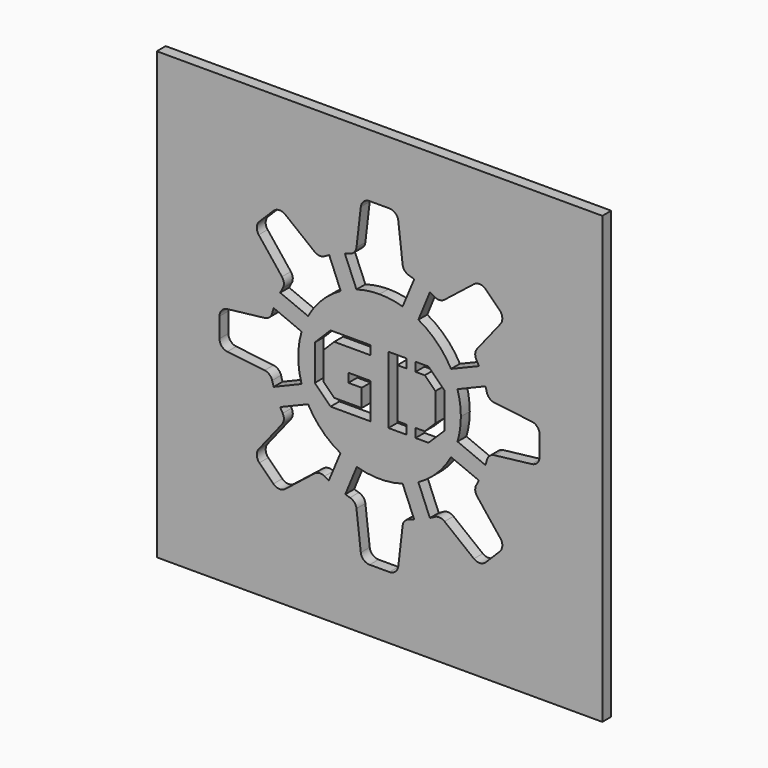
from build123d import *

# Parameters (mm, degrees)
F0_W     = 127
F0_H     = 127
F1_DEPTH = 3.175
F3_DEPTH = 3.175
F5_DEPTH = 3.175
F7_DEPTH = 3.175


with BuildPart() as f1:
    # F0 (on Front) → F1 (new body)
    with BuildSketch(Plane.XZ):
        Rectangle(F0_W, F0_H)
    extrude(amount=-F1_DEPTH)

    # F2 (on face) → F3 (cut, through all)
    with BuildSketch(Plane.XZ):
        with BuildLine():
            ThreePointArc((-6.5756926955, 32.7672866468), (-7.1708300148, 31.407037356), (-8.424698119, 30.611876153))
            ThreePointArc((-8.424698119, 30.611876153), (-12.1501989776, 29.3331751572), (-15.6887040432, 27.603026382))
            ThreePointArc((-15.6887040432, 27.603026382), (-17.1375865613, 27.2786716216), (-18.520253693, 27.819687485))
            Line((-18.520253693, 27.819687485), (-26.8947926181, 34.4486268529))
            ThreePointArc((-26.8947926181, 34.4486268529), (-28.6182622131, 34.9927875941), (-30.2672971687, 34.2530970695))
            Line((-30.2672971687, 34.2530970695), (-32.2601971191, 32.2601971191))
            Line((-32.2601971191, 32.2601971191), (-34.2530970695, 30.2672971687))
            ThreePointArc((-34.2530970695, 30.2672971687), (-34.9927875941, 28.6182622131), (-34.4486268529, 26.8947926181))
            Line((-34.4486268529, 26.8947926181), (-27.819687485, 18.520253693))
            ThreePointArc((-27.819687485, 18.520253693), (-27.2786716216, 17.1375865613), (-27.603026382, 15.6887040432))
            ThreePointArc((-27.603026382, 15.6887040432), (-29.3331751572, 12.1501989776), (-30.611876153, 8.424698119))
            ThreePointArc((-30.611876153, 8.424698119), (-31.407037356, 7.1708300148), (-32.7672866468, 6.5756926955))
            Line((-32.7672866468, 6.5756926955), (-43.3763478891, 5.3413674113))
            ThreePointArc((-43.3763478891, 5.3413674113), (-44.9798046771, 4.5074701238), (-45.6228082907, 2.8183861383))
            Line((-45.6228082907, 2.8183861383), (-45.6228082907, 0))
            Line((-45.6228082907, 0), (-45.6228082907, -2.8183861383))
            ThreePointArc((-45.6228082907, -2.8183861383), (-44.9798046771, -4.5074701238), (-43.3763478891, -5.3413674113))
            Line((-43.3763478891, -5.3413674113), (-32.7672866468, -6.5756926955))
            ThreePointArc((-32.7672866468, -6.5756926955), (-31.407037356, -7.1708300148), (-30.611876153, -8.424698119))
            ThreePointArc((-30.611876153, -8.424698119), (-29.3331751572, -12.1501989776), (-27.603026382, -15.6887040432))
            ThreePointArc((-27.603026382, -15.6887040432), (-27.2786716216, -17.1375865613), (-27.819687485, -18.520253693))
            Line((-27.819687485, -18.520253693), (-34.4486268529, -26.8947926181))
            ThreePointArc((-34.4486268529, -26.8947926181), (-34.9927875941, -28.6182622131), (-34.2530970695, -30.2672971687))
            Line((-34.2530970695, -30.2672971687), (-32.2601971191, -32.2601971191))
            Line((-32.2601971191, -32.2601971191), (-30.2672971687, -34.2530970695))
            ThreePointArc((-30.2672971687, -34.2530970695), (-28.6182622131, -34.9927875941), (-26.8947926181, -34.4486268529))
            Line((-26.8947926181, -34.4486268529), (-18.520253693, -27.819687485))
            ThreePointArc((-18.520253693, -27.819687485), (-17.1375865613, -27.2786716216), (-15.6887040432, -27.603026382))
            ThreePointArc((-15.6887040432, -27.603026382), (-15.0740522826, -27.9434329992), (-14.452018381, -28.2701550175))
            Line((-14.452018381, -28.2701550175), (-11.1423706298, -20.3234859952))
            ThreePointArc((-11.1423706298, -20.3234859952), (-22.452662458, 5.7510394537), (0, 23.1775))
            Line((0, 23.1775), (0, 45.6228082907))
            Line((0, 45.6228082907), (-2.8183861383, 45.6228082907))
            ThreePointArc((-2.8183861383, 45.6228082907), (-4.5074701238, 44.9798046771), (-5.3413674113, 43.3763478891))
            Line((-5.3413674113, 43.3763478891), (-6.5756926955, 32.7672866468))
        make_face()
        with BuildLine():
            Line((2.8183861383, 45.6228082907), (0, 45.6228082907))
            Line((0, 45.6228082907), (0, 23.1775))
            ThreePointArc((0, 23.1775), (3.3233858671, 22.9379949566), (6.578087219, 22.2244296842))
            Line((6.578087219, 22.2244296842), (9.8877349702, 30.1710987065))
            ThreePointArc((9.8877349702, 30.1710987065), (9.1588685219, 30.4002899229), (8.424698119, 30.611876153))
            ThreePointArc((8.424698119, 30.611876153), (7.1708300148, 31.407037356), (6.5756926955, 32.7672866468))
            Line((6.5756926955, 32.7672866468), (5.3413674113, 43.3763478891))
            ThreePointArc((5.3413674113, 43.3763478891), (4.5074701238, 44.9798046771), (2.8183861383, 45.6228082907))
        make_face()
        with BuildLine():
            Line((9.8877349702, 30.1710987065), (6.578087219, 22.2244296842))
            ThreePointArc((6.578087219, 22.2244296842), (7.7345087621, 21.8488873964), (8.8696452536, 21.4132178648))
            Line((8.8696452536, 21.4132178648), (12.1501989776, 29.3331751572))
            ThreePointArc((12.1501989776, 29.3331751572), (11.0269289533, 29.7736349454), (9.8877349702, 30.1710987065))
        make_face()
        with BuildLine():
            ThreePointArc((-8.8696452536, -21.4132178648), (-10.0208319922, -20.8992687057), (-11.1423706298, -20.3234859952))
            Line((-11.1423706298, -20.3234859952), (-14.452018381, -28.2701550175))
            ThreePointArc((-14.452018381, -28.2701550175), (-13.31172397, -28.8246509944), (-12.1501989776, -29.3331751572))
            Line((-12.1501989776, -29.3331751572), (-8.8696452536, -21.4132178648))
        make_face()
        with BuildLine():
            Line((12.1501989776, 29.3331751572), (8.8696452536, 21.4132178648))
            ThreePointArc((8.8696452536, 21.4132178648), (9.9803728445, 20.9186200342), (11.0636348579, 20.3664550175))
            Line((11.0636348579, 20.3664550175), (14.3425040432, 28.3258729393))
            ThreePointArc((14.3425040432, 28.3258729393), (13.2559229319, 28.850355409), (12.1501989776, 29.3331751572))
        make_face()
        with BuildLine():
            ThreePointArc((-6.4920289337, -22.2497205954), (-7.6922163688, -21.8638128785), (-8.8696452536, -21.4132178648))
            Line((-8.8696452536, -21.4132178648), (-12.1501989776, -29.3331751572))
            ThreePointArc((-12.1501989776, -29.3331751572), (-10.969295895, -29.7949164719), (-9.770898119, -30.2091385171))
            Line((-9.770898119, -30.2091385171), (-6.4920289337, -22.2497205954))
        make_face()
        with BuildLine():
            Line((14.3425040432, 28.3258729393), (11.0636348579, 20.3664550175))
            ThreePointArc((11.0636348579, 20.3664550175), (19.9201393465, 11.8483988228), (23.1775, 0))
            ThreePointArc((23.1775, 0), (13.9055295771, -18.5427277775), (-6.4920289337, -22.2497205954))
            Line((-6.4920289337, -22.2497205954), (-9.770898119, -30.2091385171))
            ThreePointArc((-9.770898119, -30.2091385171), (-9.1000263744, -30.4179555524), (-8.424698119, -30.611876153))
            ThreePointArc((-8.424698119, -30.611876153), (-7.1708300148, -31.407037356), (-6.5756926955, -32.7672866468))
            Line((-6.5756926955, -32.7672866468), (-5.3413674113, -43.3763478891))
            ThreePointArc((-5.3413674113, -43.3763478891), (-4.5074701238, -44.9798046771), (-2.8183861383, -45.6228082907))
            Line((-2.8183861383, -45.6228082907), (0, -45.6228082907))
            Line((0, -45.6228082907), (2.8183861383, -45.6228082907))
            ThreePointArc((2.8183861383, -45.6228082907), (4.5074701238, -44.9798046771), (5.3413674113, -43.3763478891))
            Line((5.3413674113, -43.3763478891), (6.5756926955, -32.7672866468))
            ThreePointArc((6.5756926955, -32.7672866468), (7.1708300148, -31.407037356), (8.424698119, -30.611876153))
            ThreePointArc((8.424698119, -30.611876153), (12.1501989776, -29.3331751572), (15.6887040432, -27.603026382))
            ThreePointArc((15.6887040432, -27.603026382), (17.1375865613, -27.2786716216), (18.520253693, -27.819687485))
            Line((18.520253693, -27.819687485), (26.8947926181, -34.4486268529))
            ThreePointArc((26.8947926181, -34.4486268529), (28.6182622131, -34.9927875941), (30.2672971687, -34.2530970695))
            Line((30.2672971687, -34.2530970695), (32.2601971191, -32.2601971191))
            Line((32.2601971191, -32.2601971191), (34.2530970695, -30.2672971687))
            ThreePointArc((34.2530970695, -30.2672971687), (34.9927875941, -28.6182622131), (34.4486268529, -26.8947926181))
            Line((34.4486268529, -26.8947926181), (27.819687485, -18.520253693))
            ThreePointArc((27.819687485, -18.520253693), (27.2786716216, -17.1375865613), (27.603026382, -15.6887040432))
            ThreePointArc((27.603026382, -15.6887040432), (29.3331751572, -12.1501989776), (30.611876153, -8.424698119))
            ThreePointArc((30.611876153, -8.424698119), (31.407037356, -7.1708300148), (32.7672866468, -6.5756926955))
            Line((32.7672866468, -6.5756926955), (43.3763478891, -5.3413674113))
            ThreePointArc((43.3763478891, -5.3413674113), (44.9798046771, -4.5074701238), (45.6228082907, -2.8183861383))
            Line((45.6228082907, -2.8183861383), (45.6228082907, 0))
            Line((45.6228082907, 0), (45.6228082907, 2.8183861383))
            ThreePointArc((45.6228082907, 2.8183861383), (44.9798046771, 4.5074701238), (43.3763478891, 5.3413674113))
            Line((43.3763478891, 5.3413674113), (32.7672866468, 6.5756926955))
            ThreePointArc((32.7672866468, 6.5756926955), (31.407037356, 7.1708300148), (30.611876153, 8.424698119))
            ThreePointArc((30.611876153, 8.424698119), (29.3331751572, 12.1501989776), (27.603026382, 15.6887040432))
            ThreePointArc((27.603026382, 15.6887040432), (27.2786716216, 17.1375865613), (27.819687485, 18.520253693))
            Line((27.819687485, 18.520253693), (34.4486268529, 26.8947926181))
            ThreePointArc((34.4486268529, 26.8947926181), (34.9927875941, 28.6182622131), (34.2530970695, 30.2672971687))
            Line((34.2530970695, 30.2672971687), (32.2601971191, 32.2601971191))
            Line((32.2601971191, 32.2601971191), (30.2672971687, 34.2530970695))
            ThreePointArc((30.2672971687, 34.2530970695), (28.6182622131, 34.9927875941), (26.8947926181, 34.4486268529))
            Line((26.8947926181, 34.4486268529), (18.520253693, 27.819687485))
            ThreePointArc((18.520253693, 27.819687485), (17.1375865613, 27.2786716216), (15.6887040432, 27.603026382))
            ThreePointArc((15.6887040432, 27.603026382), (15.0199531147, 27.9725491944), (14.3425040432, 28.3258729393))
        make_face()
    extrude(amount=-F3_DEPTH, mode=Mode.SUBTRACT)

    # F4 (on face) → F5 (join, through all)
    with BuildSketch(Plane.XZ):
        Polygon((11.0636348579, 20.3664550175), (14.3425040432, 28.3258729393), (14.3425040432, 32.367836684), (9.8877349702, 30.1710987065), (6.578087219, 22.2244296842), (6.578087219, 19.2353967577), align=None)
        Polygon((-9.770898119, -30.2091385171), (-6.4920289337, -22.2497205954), (-6.578087219, -21.9381616706), (-6.578087219, -22.2244296842), (-9.8877349702, -30.1710987065), (-13.9834821743, -32.1907956385), (-13.8441137969, -33.3570092916), align=None)
        Polygon((-6.578087219, -22.2244296842), (-6.578087219, -21.9381616706), (-7.2760287021, -19.4113869696), (-11.0636348579, -20.3664550175), (-14.3425040432, -28.3258729393), (-14.3425040432, -29.1865545515), (-13.9834821743, -32.1907956385), (-9.8877349702, -30.1710987065), align=None)
        Polygon((-7.2760287021, -19.4113869696), (-6.578087219, -21.9381616706), (-6.578087219, -19.2353967577), align=None)
        Polygon((-11.0636348579, -20.3664550175), (-7.2760287021, -19.4113869696), (-7.9609118402, -16.9318877161), (-11.1423706298, -20.3234859952), (-14.452018381, -28.2701550175), (-14.3425040432, -29.1865545515), (-14.3425040432, -28.3258729393), align=None)
        Polygon((-14.3425040432, -32.367836684), (-13.9834821743, -32.1907956385), (-14.3425040432, -29.1865545515), align=None)
        Polygon((-12.7458349434, 33.0291986797), (-14.3425040432, 28.3258729393), (-11.0636348579, 20.3664550175), (-8.9500694064, 18.252889566), (-6.578087219, 22.2244296842), (-9.8877349702, 30.1710987065), align=None)
        Polygon((-32.367836684, 14.3425040432), (-30.1710987065, 9.8877349702), (-22.2244296842, 6.578087219), (-19.2353967577, 6.578087219), (-20.3664550175, 11.0636348579), (-28.3258729393, 14.3425040432), align=None)
        Polygon((-33.0291986797, -12.7458349434), (-28.3258729393, -14.3425040432), (-20.3664550175, -11.0636348579), (-18.252889566, -8.9500694064), (-22.2244296842, -6.578087219), (-30.1710987065, -9.8877349702), align=None)
        Polygon((12.7458349434, -33.0291986797), (14.3425040432, -28.3258729393), (11.0636348579, -20.3664550175), (8.9500694064, -18.252889566), (6.578087219, -22.2244296842), (9.8877349702, -30.1710987065), align=None)
        Polygon((32.367836684, -14.3425040432), (30.1710987065, -9.8877349702), (22.2244296842, -6.578087219), (19.2353967577, -6.578087219), (20.3664550175, -11.0636348579), (28.3258729393, -14.3425040432), align=None)
        Polygon((33.0291986797, 12.7458349434), (28.3258729393, 14.3425040432), (20.3664550175, 11.0636348579), (18.252889566, 8.9500694064), (22.2244296842, 6.578087219), (30.1710987065, 9.8877349702), align=None)
    extrude(amount=-F5_DEPTH)

    # F6 (on face) → F7 (cut, through all)
    with BuildSketch(Plane.XZ):
        Polygon((-2.54, 7.0301280605), (-2.54, 9.5701280605), (-13.97, 9.5701280605), (-18.4601280605, 5.08), (-18.4601280605, -5.08), (-13.97, -9.5701280605), (-2.54, -9.5701280605), (-2.54, -7.0301280605), (-2.54, 0.5898719395), (-8.89, 0.5898719395), (-8.89, -1.9501280605), (-5.08, -1.9501280605), (-5.08, -7.0301280605), (-12.9178975516, -7.0301280605), (-15.9201280605, -4.0278975516), (-15.9201280605, 4.0278975516), (-12.9178975516, 7.0301280605), align=None)
        Polygon((7.7216, 9.5701280605), (2.54, 9.5701280605), (2.54, -9.5701280605), (7.7216, -9.5701280605), (7.7216, -7.0301280605), (5.08, -7.0301280605), (5.08, 7.0301280605), (7.7216, 7.0301280605), align=None)
        Polygon((10.2616, -9.5701280605), (13.9451769065, -9.5701280605), (18.4658, -5.1107035633), (18.4658, 0), (18.4658, 5.1107035633), (13.9451769065, 9.5701280605), (10.2616, 9.5701280605), (10.2616, 7.0301280605), (12.9032, 7.0301280605), (15.9258, 4.04844695), (15.9258, 0), (15.9258, -4.04844695), (12.9032, -7.0301280605), (10.2616, -7.0301280605), align=None)
    extrude(amount=-F7_DEPTH, mode=Mode.SUBTRACT)


solid = f1.part
